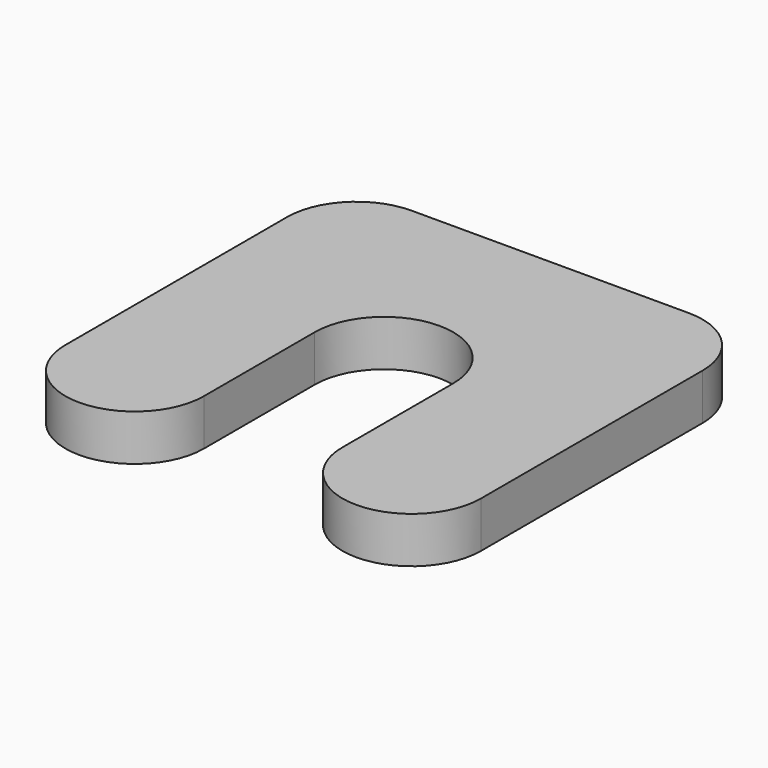
from build123d import *

# Parameters (mm, degrees)
F1_DEPTH     = 10
F2_T         = -2.5
F3_TEXT_SIZE = 5.7622764467
F4_DEPTH     = 2.5


# Not quite as in the source:
# - Text() gives the source's letters only with a copy of the font that has no kerning and outlines rounded to 1/6400 em; it was checked with that copy


with BuildPart() as f1:
    # F0 (on Top) → F1 (new body)
    with BuildSketch(Plane.XY):
        with BuildLine():
            Line((31.1277738959, 30), (-28.8722261041, 30))
            ThreePointArc((-28.8722261041, 30), (-39.4788278219, 25.6066017178), (-43.8722261041, 15))
            Line((-43.8722261041, 15), (-43.8722261041, -45))
            ThreePointArc((-43.8722261041, -45), (-39.4788278219, -55.6066017178), (-28.8722261041, -60))
            ThreePointArc((-28.8722261041, -60), (-18.2656243863, -55.6066017178), (-13.8722261041, -45))
            Line((-13.8722261041, -45), (-13.8722261041, -15))
            ThreePointArc((-13.8722261041, -15), (-9.4788278219, -4.3933982822), (1.1277738959, 0))
            ThreePointArc((1.1277738959, 0), (11.7343756137, -4.3933982822), (16.1277738959, -15))
            Line((16.1277738959, -15), (16.1277738959, -45))
            ThreePointArc((16.1277738959, -45), (20.5211721781, -55.6066017178), (31.1277738959, -60))
            ThreePointArc((31.1277738959, -60), (41.7343756137, -55.6066017178), (46.1277738959, -45))
            Line((46.1277738959, -45), (46.1277738959, 15))
            ThreePointArc((46.1277738959, 15), (41.7343756137, 25.6066017178), (31.1277738959, 30))
        make_face()
    extrude(amount=F1_DEPTH)

    # F2
    f2_openings = [f1.faces().sort_by_distance(p)[0] for p in [
        (-38.578828, 24.706602, 0),
    ]]
    offset(amount=F2_T, openings=f2_openings)

    # F3 (on face) → F4 (join)
    with BuildSketch(Plane(origin=(0, 0, 7.5), x_dir=(1, 0, 0), z_dir=(0, 0, -1))):
        with Locations((-2.0500160754, -20.6645131111)):
            Text('Raquel', F3_TEXT_SIZE, font='Open Sans', text_align=(TextAlign.LEFT, TextAlign.BOTTOM))
    extrude(amount=F4_DEPTH)


solid = f1.part
